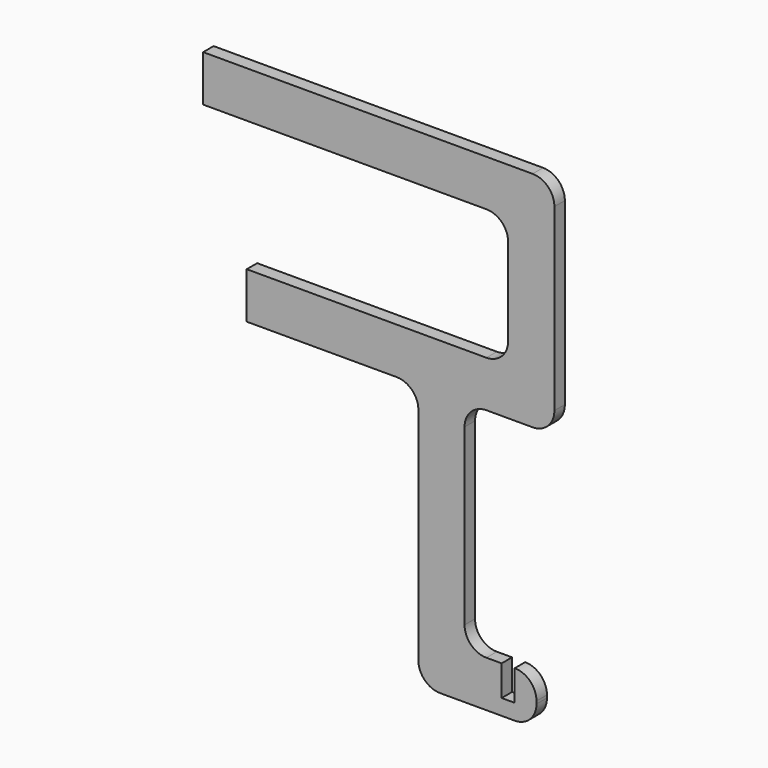
from build123d import *

# Parameters (mm, degrees)
F1_DEPTH = 3
F2_R     = 4.99999


# Not quite as in the source:
# - a fillet or chamfer is up to 0.001 mm smaller than in the source, because OpenCascade refuses the exact size


with BuildPart() as f1:
    # F0 (on Front) → F1 (new body)
    with BuildSketch(Plane.XZ):
        Polygon((80.6066017178, 0), (0, 0), (0, -10.6066017178), (70, -10.6066017178), (70, -40.6066017178), (10, -40.6066017178), (10, -51.2132034356), (49.3933982822, -51.2132034356), (49.3933982822, -111.8198051534), (76.5, -111.8198051534), (76.5, -101.2132034356), (71.5, -101.2132034356), (71.5, -108.2132034356), (68.5, -108.2132034356), (68.5, -101.2132034356), (60, -101.2132034356), (60, -51.2132034356), (80.6066017178, -51.2132034356), align=None)
    extrude(amount=F1_DEPTH)

    # F2 (radius 5 in the source; OpenCascade refuses exactly that, so slightly less here)
    f2_edges = [f1.edges().sort_by_distance(p)[0] for p in [
        (49.393398, -1.5, -51.213203),
        (70, -1.5, -10.606602),
        (70, -1.5, -40.606602),
        (80.606602, -1.5, 0),
        (80.606602, -1.5, -51.213203),
        (60, -1.5, -51.213203),
        (60, -1.5, -101.213203),
        (76.5, -1.5, -101.213203),
        (76.5, -1.5, -111.819805),
        (49.393398, -1.5, -111.819805),
    ]]
    fillet(f2_edges, radius=F2_R)


solid = f1.part
